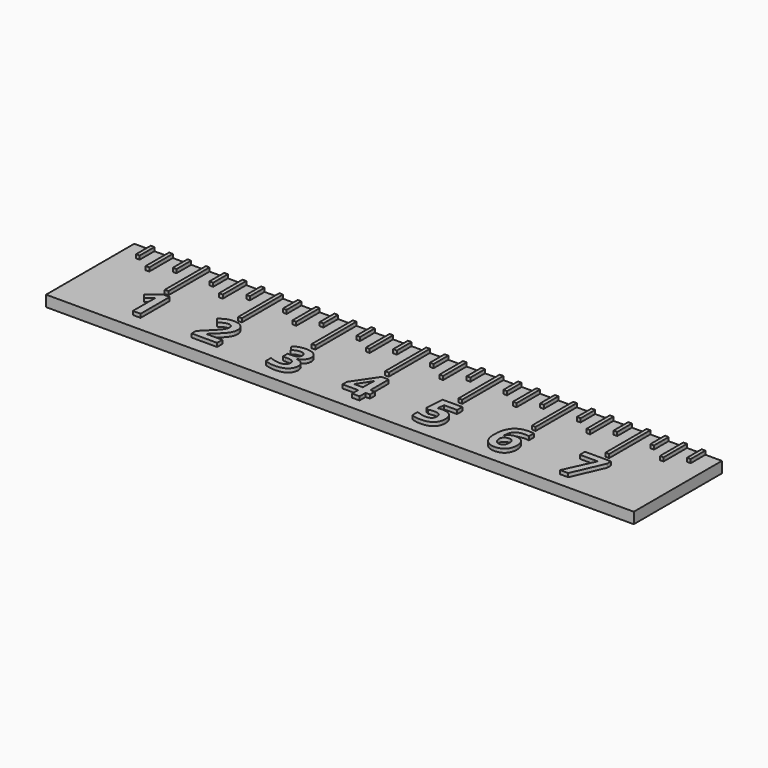
from build123d import *

# Parameters (mm, degrees)
F1_DEPTH     = 3.81
F0_W         = 0.635
F0_H         = 6.35
F0_H_2       = 10.16
F0_H_3       = 17.78
F0_TEXT_SIZE = 17.6388888889
F2_DEPTH     = 5.08


# Not quite as in the source:
# - Text() gives the source's letters only with a copy of the font that has no kerning and outlines rounded to 1/6400 em; it was checked with that copy


with BuildPart() as f1:
    # F0 (on Top) → F1 (new body)
    with BuildSketch(Plane.XY):
        Polygon((-69.85, 29.4929609475), (-75.565, 29.4929609475), (-75.565, -8.6070390525), (127.635, -8.6070390525), (127.635, 29.4929609475), (121.92, 29.4929609475), (121.92, 23.1429609475), (121.285, 23.1429609475), (120.65, 23.1429609475), (120.65, 29.4929609475), (115.57, 29.4929609475), (115.57, 19.3329609475), (114.935, 19.3329609475), (114.3, 19.3329609475), (114.3, 29.4929609475), (109.22, 29.4929609475), (109.22, 23.1429609475), (108.585, 23.1429609475), (107.95, 23.1429609475), (107.95, 29.4929609475), (102.87, 29.4929609475), (102.87, 11.7129609475), (102.235, 11.7129609475), (101.6, 11.7129609475), (101.6, 29.4929609475), (96.52, 29.4929609475), (96.52, 23.1429609475), (95.885, 23.1429609475), (95.25, 23.1429609475), (95.25, 29.4929609475), (90.17, 29.4929609475), (90.17, 19.3329609475), (89.535, 19.3329609475), (88.9, 19.3329609475), (88.9, 29.4929609475), (83.82, 29.4929609475), (83.82, 23.1429609475), (83.185, 23.1429609475), (82.55, 23.1429609475), (82.55, 29.4929609475), (77.47, 29.4929609475), (77.47, 11.7129609475), (76.835, 11.7129609475), (76.2, 11.7129609475), (76.2, 29.4929609475), (71.12, 29.4929609475), (71.12, 23.1429609475), (70.485, 23.1429609475), (69.85, 23.1429609475), (69.85, 29.4929609475), (64.77, 29.4929609475), (64.77, 19.3329609475), (64.135, 19.3329609475), (63.5, 19.3329609475), (63.5, 29.4929609475), (58.42, 29.4929609475), (58.42, 23.1429609475), (57.785, 23.1429609475), (57.15, 23.1429609475), (57.15, 29.4929609475), (52.07, 29.4929609475), (52.07, 11.7129609475), (51.435, 11.7129609475), (50.8, 11.7129609475), (50.8, 29.4929609475), (45.72, 29.4929609475), (45.72, 23.1429609475), (45.085, 23.1429609475), (44.45, 23.1429609475), (44.45, 29.4929609475), (39.37, 29.4929609475), (39.37, 19.3329609475), (38.735, 19.3329609475), (38.1, 19.3329609475), (38.1, 29.4929609475), (33.02, 29.4929609475), (33.02, 23.1429609475), (32.385, 23.1429609475), (31.75, 23.1429609475), (31.75, 29.4929609475), (26.67, 29.4929609475), (26.67, 11.7129609475), (26.035, 11.7129609475), (25.4, 11.7129609475), (25.4, 29.4929609475), (20.32, 29.4929609475), (20.32, 23.1429609475), (19.685, 23.1429609475), (19.05, 23.1429609475), (19.05, 29.4929609475), (13.97, 29.4929609475), (13.97, 19.3329609475), (13.335, 19.3329609475), (12.7, 19.3329609475), (12.7, 29.4929609475), (7.62, 29.4929609475), (7.62, 23.1429609475), (6.985, 23.1429609475), (6.35, 23.1429609475), (6.35, 29.4929609475), (1.27, 29.4929609475), (1.27, 11.7129609475), (0.635, 11.7129609475), (0, 11.7129609475), (0, 29.4929609475), (-5.08, 29.4929609475), (-5.08, 23.1429609475), (-5.715, 23.1429609475), (-6.35, 23.1429609475), (-6.35, 29.4929609475), (-11.43, 29.4929609475), (-11.43, 19.3329609475), (-12.065, 19.3329609475), (-12.7, 19.3329609475), (-12.7, 29.4929609475), (-17.78, 29.4929609475), (-17.78, 23.1429609475), (-18.415, 23.1429609475), (-19.05, 23.1429609475), (-19.05, 29.4929609475), (-24.13, 29.4929609475), (-24.13, 11.7129609475), (-24.765, 11.7129609475), (-25.4, 11.7129609475), (-25.4, 29.4929609475), (-30.48, 29.4929609475), (-30.48, 23.1429609475), (-31.115, 23.1429609475), (-31.75, 23.1429609475), (-31.75, 29.4929609475), (-36.83, 29.4929609475), (-36.83, 19.3329609475), (-37.465, 19.3329609475), (-38.1, 19.3329609475), (-38.1, 29.4929609475), (-43.18, 29.4929609475), (-43.18, 23.1429609475), (-43.815, 23.1429609475), (-44.45, 23.1429609475), (-44.45, 29.4929609475), (-49.53, 29.4929609475), (-49.53, 11.7129609475), (-50.165, 11.7129609475), (-50.8, 11.7129609475), (-50.8, 29.4929609475), (-55.88, 29.4929609475), (-55.88, 23.1429609475), (-56.515, 23.1429609475), (-57.15, 23.1429609475), (-57.15, 29.4929609475), (-62.23, 29.4929609475), (-62.23, 19.3329609475), (-62.865, 19.3329609475), (-63.5, 19.3329609475), (-63.5, 29.4929609475), (-68.58, 29.4929609475), (-68.58, 23.1429609475), (-69.215, 23.1429609475), (-69.85, 23.1429609475), align=None)
        with BuildLine():
            Line((-47.136638159, 9.3029846763), (-47.136638159, -3.2895283446))
            Line((-47.136638159, -3.2895283446), (-49.7990079507, -3.2895283446))
            Line((-49.7990079507, -3.2895283446), (-49.7990079507, 3.9975376277))
            Line((-49.7990079507, 3.9975376277), (-49.7714471868, 5.1936747804))
            Line((-49.7714471868, 5.1936747804), (-49.7301060409, 6.5028110652))
            add(Edge.make_bspline(
                [(-49.7301060409, 6.5028110652), (-50.3915643743, 5.8413527318), (-50.6506355548, 5.6346470027)],
                knots=[0, 0, 0, 1, 1, 1], degree=2))
            Line((-50.6506355548, 5.6346470027), (-52.097575659, 4.4715827665))
            Line((-52.097575659, 4.4715827665), (-53.3819072562, 6.0728631485))
            Line((-53.3819072562, 6.0728631485), (-49.3249628118, 9.3029846763))
            Line((-49.3249628118, 9.3029846763), (-47.136638159, 9.3029846763))
        make_face(mode=Mode.SUBTRACT)
        with BuildLine():
            Line((-20.3797193368, -1.4265028158), (-20.3797193368, -3.6671929199))
            Line((-20.3797193368, -3.6671929199), (-29.1826273229, -3.6671929199))
            Line((-29.1826273229, -3.6671929199), (-29.1826273229, -1.8151095866))
            Line((-29.1826273229, -1.8151095866), (-26.0214077049, 1.3791829481))
            add(Edge.make_bspline(
                [(-26.0214077049, 1.3791829481), (-24.6158087465, 2.8178548231), (-24.1858608299, 3.3732042155)],
                knots=[0, 0, 0, 1, 1, 1], degree=2))
            add(Edge.make_bspline(
                [(-24.1858608299, 3.3732042155), (-23.7559129132, 3.9285536079), (-23.5657436424, 4.4025987467)],
                knots=[0, 0, 0, 1, 1, 1], degree=2))
            add(Edge.make_bspline(
                [(-23.5657436424, 4.4025987467), (-23.3755743715, 4.8766438856), (-23.3755743715, 5.3837619412)],
                knots=[0, 0, 0, 1, 1, 1], degree=2))
            add(Edge.make_bspline(
                [(-23.3755743715, 5.3837619412), (-23.3755743715, 6.1416829481), (-23.7944979827, 6.5123752224)],
                knots=[0, 0, 0, 1, 1, 1], degree=2))
            add(Edge.make_bspline(
                [(-23.7944979827, 6.5123752224), (-24.2134215938, 6.8830674967), (-24.9107089202, 6.8830674967)],
                knots=[0, 0, 0, 1, 1, 1], degree=2))
            add(Edge.make_bspline(
                [(-24.9107089202, 6.8830674967), (-25.6410691632, 6.8830674967), (-26.3300882604, 6.5468261773)],
                knots=[0, 0, 0, 1, 1, 1], degree=2))
            add(Edge.make_bspline(
                [(-26.3300882604, 6.5468261773), (-27.0191073577, 6.2105848579), (-27.7687601354, 5.5904676704)],
                knots=[0, 0, 0, 1, 1, 1], degree=2))
            Line((-27.7687601354, 5.5904676704), (-29.2157002396, 7.3047471842))
            add(Edge.make_bspline(
                [(-29.2157002396, 7.3047471842), (-28.2869024965, 8.0984971842), (-27.6750535382, 8.4250922363)],
                knots=[0, 0, 0, 1, 1, 1], degree=2))
            add(Edge.make_bspline(
                [(-27.6750535382, 8.4250922363), (-27.0632045799, 8.7516872884), (-26.3397345278, 8.9280761773)],
                knots=[0, 0, 0, 1, 1, 1], degree=2))
            add(Edge.make_bspline(
                [(-26.3397345278, 8.9280761773), (-25.6162644757, 9.1044650662), (-24.7205396493, 9.1044650662)],
                knots=[0, 0, 0, 1, 1, 1], degree=2))
            add(Edge.make_bspline(
                [(-24.7205396493, 9.1044650662), (-23.5409389549, 9.1044650662), (-22.6369458993, 8.6745171495)],
                knots=[0, 0, 0, 1, 1, 1], degree=2))
            add(Edge.make_bspline(
                [(-22.6369458993, 8.6745171495), (-21.7329528438, 8.2445692329), (-21.2327249792, 7.4687337294)],
                knots=[0, 0, 0, 1, 1, 1], degree=2))
            add(Edge.make_bspline(
                [(-21.2327249792, 7.4687337294), (-20.7324971146, 6.6928982259), (-20.7324971146, 5.6951985731)],
                knots=[0, 0, 0, 1, 1, 1], degree=2))
            add(Edge.make_bspline(
                [(-20.7324971146, 5.6951985731), (-20.7324971146, 4.8242784342), (-21.0384215938, 4.0622233127)],
                knots=[0, 0, 0, 1, 1, 1], degree=2))
            add(Edge.make_bspline(
                [(-21.0384215938, 4.0622233127), (-21.3443460729, 3.3001681912), (-21.9865118715, 2.4995280002)],
                knots=[0, 0, 0, 1, 1, 1], degree=2))
            add(Edge.make_bspline(
                [(-21.9865118715, 2.4995280002), (-22.6286776702, 1.6988878092), (-24.2464945104, 0.216118712)],
                knots=[0, 0, 0, 1, 1, 1], degree=2))
            Line((-24.2464945104, 0.216118712), (-25.8670674271, -1.307991531))
            Line((-25.8670674271, -1.307991531), (-25.8670674271, -1.4265028158))
            Line((-25.8670674271, -1.4265028158), (-20.3797193368, -1.4265028158))
        make_face(mode=Mode.SUBTRACT)
        with BuildLine():
            add(Edge.make_bspline(
                [(3.7243620052, 7.7445760939), (4.857109401, 6.9522041321), (4.857109401, 5.541093021)],
                knots=[0, 0, 0, 1, 1, 1], degree=2))
            add(Edge.make_bspline(
                [(4.857109401, 5.541093021), (4.857109401, 4.3614923265), (4.1419075781, 3.5346694099)],
                knots=[0, 0, 0, 1, 1, 1], degree=2))
            add(Edge.make_bspline(
                [(4.1419075781, 3.5346694099), (3.4267057552, 2.7078464932), (2.1341059288, 2.3964098612)],
                knots=[0, 0, 0, 1, 1, 1], degree=2))
            Line((2.1341059288, 2.3964098612), (2.1341059288, 2.3468004862))
            add(Edge.make_bspline(
                [(2.1341059288, 2.3468004862), (3.6609722483, 2.1566312154), (4.4436979427, 1.4193807814)],
                knots=[0, 0, 0, 1, 1, 1], degree=2))
            add(Edge.make_bspline(
                [(4.4436979427, 1.4193807814), (5.2264236372, 0.6821303474), (5.2264236372, -0.5663722568)],
                knots=[0, 0, 0, 1, 1, 1], degree=2))
            add(Edge.make_bspline(
                [(5.2264236372, -0.5663722568), (5.2264236372, -2.3826265971), (3.9090191233, -3.39548467)],
                knots=[0, 0, 0, 1, 1, 1], degree=2))
            add(Edge.make_bspline(
                [(3.9090191233, -3.39548467), (2.5916146094, -4.4083427429), (0.1469748524, -4.4083427429)],
                knots=[0, 0, 0, 1, 1, 1], degree=2))
            add(Edge.make_bspline(
                [(0.1469748524, -4.4083427429), (-1.9035459809, -4.4083427429), (-3.4882899045, -3.7275918749)],
                knots=[0, 0, 0, 1, 1, 1], degree=2))
            Line((-3.4882899045, -3.7275918749), (-3.4882899045, -1.4620970832))
            add(Edge.make_bspline(
                [(-3.4882899045, -1.4620970832), (-2.7579296615, -1.8314113193), (-1.8787412934, -2.0642997742)],
                knots=[0, 0, 0, 1, 1, 1], degree=2))
            add(Edge.make_bspline(
                [(-1.8787412934, -2.0642997742), (-0.9995529253, -2.297188229), (-0.139657092, -2.297188229)],
                knots=[0, 0, 0, 1, 1, 1], degree=2))
            add(Edge.make_bspline(
                [(-0.139657092, -2.297188229), (1.1805034983, -2.297188229), (1.8088889149, -1.8493258158)],
                knots=[0, 0, 0, 1, 1, 1], degree=2))
            add(Edge.make_bspline(
                [(1.8088889149, -1.8493258158), (2.4372743316, -1.4014634026), (2.4372743316, -0.4092759026)],
                knots=[0, 0, 0, 1, 1, 1], degree=2))
            add(Edge.make_bspline(
                [(2.4372743316, -0.4092759026), (2.4372743316, 0.4754246182), (1.7138042795, 0.8461168925)],
                knots=[0, 0, 0, 1, 1, 1], degree=2))
            add(Edge.make_bspline(
                [(1.7138042795, 0.8461168925), (0.9903342274, 1.2168091668), (-0.5944096962, 1.2168091668)],
                knots=[0, 0, 0, 1, 1, 1], degree=2))
            Line((-0.5944096962, 1.2168091668), (-1.5507682031, 1.2168091668))
            Line((-1.5507682031, 1.2168091668), (-1.5507682031, 3.259061771))
            Line((-1.5507682031, 3.259061771), (-0.5778732378, 3.259061771))
            add(Edge.make_bspline(
                [(-0.5778732378, 3.259061771), (0.8856033247, 3.259061771), (1.5622200781, 3.642156389)],
                knots=[0, 0, 0, 1, 1, 1], degree=2))
            add(Edge.make_bspline(
                [(1.5622200781, 3.642156389), (2.2388368316, 4.0252510071), (2.2388368316, 4.9540487501)],
                knots=[0, 0, 0, 1, 1, 1], degree=2))
            add(Edge.make_bspline(
                [(2.2388368316, 4.9540487501), (2.2388368316, 6.384452396), (0.4473871788, 6.384452396)],
                knots=[0, 0, 0, 1, 1, 1], degree=2))
            add(Edge.make_bspline(
                [(0.4473871788, 6.384452396), (-0.1727300087, 6.384452396), (-0.8148958073, 6.1777466668)],
                knots=[0, 0, 0, 1, 1, 1], degree=2))
            add(Edge.make_bspline(
                [(-0.8148958073, 6.1777466668), (-1.4570616059, 5.9710409376), (-2.2397873003, 5.4639228821)],
                knots=[0, 0, 0, 1, 1, 1], degree=2))
            Line((-2.2397873003, 5.4639228821), (-3.4717534462, 7.2967136807))
            add(Edge.make_bspline(
                [(-3.4717534462, 7.2967136807), (-1.7492057031, 8.5369480557), (0.6375564497, 8.5369480557)],
                knots=[0, 0, 0, 1, 1, 1], degree=2))
            add(Edge.make_bspline(
                [(0.6375564497, 8.5369480557), (2.5916146094, 8.5369480557), (3.7243620052, 7.7445760939)],
                knots=[0, 0, 0, 1, 1, 1], degree=2))
        make_face(mode=Mode.SUBTRACT)
        Polygon((30.7129252507, 0.6035627079), (30.7129252507, -1.4634945838), (29.1970832368, -1.4634945838), (29.1970832368, -4.0734989241), (26.5953471257, -4.0734989241), (26.5953471257, -1.4634945838), (21.2209981673, -1.4634945838), (21.2209981673, 0.3885887495), (26.7441752507, 8.5190140968), (29.1970832368, 8.5190140968), (29.1970832368, 0.6035627079), align=None, mode=Mode.SUBTRACT)
        with BuildLine():
            add(Edge.make_bspline(
                [(50.3075025767, 3.7392927248), (50.8339131669, 3.8605600859), (51.6083706322, 3.8605600859)],
                knots=[0, 0, 0, 1, 1, 1], degree=2))
            add(Edge.make_bspline(
                [(51.6083706322, 3.8605600859), (53.4328932017, 3.8605600859), (54.5146531843, 2.8352996692)],
                knots=[0, 0, 0, 1, 1, 1], degree=2))
            add(Edge.make_bspline(
                [(54.5146531843, 2.8352996692), (55.5964131669, 1.8100392525), (55.5964131669, 0.0268578289)],
                knots=[0, 0, 0, 1, 1, 1], degree=2))
            add(Edge.make_bspline(
                [(55.5964131669, 0.0268578289), (55.5964131669, -2.0815406086), (54.2955451114, -3.2198001572)],
                knots=[0, 0, 0, 1, 1, 1], degree=2))
            add(Edge.make_bspline(
                [(54.2955451114, -3.2198001572), (52.9946770558, -4.3580597058), (50.5748419864, -4.3580597058)],
                knots=[0, 0, 0, 1, 1, 1], degree=2))
            add(Edge.make_bspline(
                [(50.5748419864, -4.3580597058), (48.4719557017, -4.3580597058), (47.1821119517, -3.6773088377)],
                knots=[0, 0, 0, 1, 1, 1], degree=2))
            Line((47.1821119517, -3.6773088377), (47.1821119517, -1.375985053))
            add(Edge.make_bspline(
                [(47.1821119517, -1.375985053), (47.8601067433, -1.73703106), (48.7654778371, -1.9657854002)],
                knots=[0, 0, 0, 1, 1, 1], degree=2))
            add(Edge.make_bspline(
                [(48.7654778371, -1.9657854002), (49.6708489308, -2.1945397405), (50.4783793128, -2.1945397405)],
                knots=[0, 0, 0, 1, 1, 1], degree=2))
            add(Edge.make_bspline(
                [(50.4783793128, -2.1945397405), (52.9175069169, -2.1945397405), (52.9175069169, -0.1963843586)],
                knots=[0, 0, 0, 1, 1, 1], degree=2))
            add(Edge.make_bspline(
                [(52.9175069169, -0.1963843586), (52.9175069169, 1.7080644262), (50.3929409447, 1.7080644262)],
                knots=[0, 0, 0, 1, 1, 1], degree=2))
            add(Edge.make_bspline(
                [(50.3929409447, 1.7080644262), (49.9381883406, 1.7080644262), (49.3869730628, 1.6171139053)],
                knots=[0, 0, 0, 1, 1, 1], degree=2))
            add(Edge.make_bspline(
                [(49.3869730628, 1.6171139053), (48.835757785, 1.5261633845), (48.4912482364, 1.4214324817)],
                knots=[0, 0, 0, 1, 1, 1], degree=2))
            Line((48.4912482364, 1.4214324817), (47.4301588267, 1.9919402942))
            Line((47.4301588267, 1.9919402942), (47.9042039656, 8.4080861275))
            Line((47.9042039656, 8.4080861275), (54.7337612572, 8.4080861275))
            Line((54.7337612572, 8.4080861275), (54.7337612572, 6.150859565))
            Line((54.7337612572, 6.150859565), (50.2386006669, 6.150859565))
            Line((50.2386006669, 6.150859565), (50.0070902503, 3.6786590442))
            Line((50.0070902503, 3.6786590442), (50.3075025767, 3.7392927248))
        make_face(mode=Mode.SUBTRACT)
        with BuildLine():
            add(Edge.make_bspline(
                [(72.0270052565, -1.835879369), (71.463387635, -0.595644994), (71.463387635, 1.1544635129)],
                knots=[0, 0, 0, 1, 1, 1], degree=2))
            add(Edge.make_bspline(
                [(71.463387635, 1.1544635129), (71.463387635, 4.8917030963), (73.043997444, 6.7176037039)],
                knots=[0, 0, 0, 1, 1, 1], degree=2))
            add(Edge.make_bspline(
                [(73.043997444, 6.7176037039), (74.624607253, 8.5435043116), (77.7775586419, 8.5435043116)],
                knots=[0, 0, 0, 1, 1, 1], degree=2))
            add(Edge.make_bspline(
                [(77.7775586419, 8.5435043116), (78.8524284336, 8.5435043116), (79.4642773919, 8.4139687213)],
                knots=[0, 0, 0, 1, 1, 1], degree=2))
            Line((79.4642773919, 8.4139687213), (79.4642773919, 6.2862777491))
            add(Edge.make_bspline(
                [(79.4642773919, 6.2862777491), (78.6980881558, 6.4599105616), (77.948435378, 6.4599105616)],
                knots=[0, 0, 0, 1, 1, 1], degree=2))
            add(Edge.make_bspline(
                [(77.948435378, 6.4599105616), (76.5786654128, 6.4599105616), (75.7132574266, 6.0464991032)],
                knots=[0, 0, 0, 1, 1, 1], degree=2))
            add(Edge.make_bspline(
                [(75.7132574266, 6.0464991032), (74.8478494405, 5.6330876449), (74.4179015239, 4.8228011866)],
                knots=[0, 0, 0, 1, 1, 1], degree=2))
            add(Edge.make_bspline(
                [(74.4179015239, 4.8228011866), (73.9879536072, 4.0125147282), (73.9107834683, 2.5242334782)],
                knots=[0, 0, 0, 1, 1, 1], degree=2))
            Line((73.9107834683, 2.5242334782), (74.0210265239, 2.5242334782))
            add(Edge.make_bspline(
                [(74.0210265239, 2.5242334782), (74.8754102044, 3.9877100407), (76.7522982253, 3.9877100407)],
                knots=[0, 0, 0, 1, 1, 1], degree=2))
            add(Edge.make_bspline(
                [(76.7522982253, 3.9877100407), (78.4390169753, 3.9877100407), (79.3953754822, 2.9279986692)],
                knots=[0, 0, 0, 1, 1, 1], degree=2))
            add(Edge.make_bspline(
                [(79.3953754822, 2.9279986692), (80.3517339891, 1.8682872977), (80.3517339891, -0.000332494)],
                knots=[0, 0, 0, 1, 1, 1], degree=2))
            add(Edge.make_bspline(
                [(80.3517339891, -0.000332494), (80.3517339891, -2.0150243343), (79.2148524787, -3.1918689523)],
                knots=[0, 0, 0, 1, 1, 1], degree=2))
            add(Edge.make_bspline(
                [(79.2148524787, -3.1918689523), (78.0779709683, -4.3687135704), (76.063279128, -4.3687135704)],
                knots=[0, 0, 0, 1, 1, 1], degree=2))
            add(Edge.make_bspline(
                [(76.063279128, -4.3687135704), (74.6687044753, -4.3687135704), (73.6296636766, -3.7224136572)],
                knots=[0, 0, 0, 1, 1, 1], degree=2))
            add(Edge.make_bspline(
                [(73.6296636766, -3.7224136572), (72.590622878, -3.076113744), (72.0270052565, -1.835879369)],
                knots=[0, 0, 0, 1, 1, 1], degree=2))
        make_face(mode=Mode.SUBTRACT)
        Polygon((101.217452068, -3.9223459687), (98.4255466861, -3.9223459687), (103.1549737694, 6.4129404896), (96.9455336652, 6.4129404896), (96.9455336652, 8.6536305938), (105.979952068, 8.6536305938), (105.979952068, 6.9806922257), align=None, mode=Mode.SUBTRACT)
    extrude(amount=F1_DEPTH)


with BuildPart() as f1b:
    # F0 (on Top) → F1, piece 2 (new body)
    with BuildSketch(Plane.XY):
        with BuildLine():
            Line((23.5636630979, 0.6035627079), (26.5953471257, 0.6035627079))
            Line((26.5953471257, 0.6035627079), (26.5953471257, 2.7395219093))
            add(Edge.make_bspline(
                [(26.5953471257, 2.7395219093), (26.5953471257, 3.2742007287), (26.6394443479, 4.289814878)],
                knots=[0, 0, 0, 1, 1, 1], degree=2))
            add(Edge.make_bspline(
                [(26.6394443479, 4.289814878), (26.6835415701, 5.3054290273), (26.7083462576, 5.4707936106)],
                knots=[0, 0, 0, 1, 1, 1], degree=2))
            Line((26.7083462576, 5.4707936106), (26.6394443479, 5.4707936106))
            add(Edge.make_bspline(
                [(26.6394443479, 5.4707936106), (26.3197394868, 4.7624819787), (25.8732551118, 4.0927554162)],
                knots=[0, 0, 0, 1, 1, 1], degree=2))
            Line((25.8732551118, 4.0927554162), (23.5636630979, 0.6035627079))
        make_face()
    extrude(amount=F1_DEPTH)


with BuildPart() as f1c:
    # F0 (on Top) → F1, piece 3 (new body)
    with BuildSketch(Plane.XY):
        with BuildLine():
            add(Edge.make_bspline(
                [(74.6452778259, -1.5340890044), (75.18409076, -2.2410225982), (76.0109136766, -2.2410225982)],
                knots=[0, 0, 0, 1, 1, 1], degree=2))
            add(Edge.make_bspline(
                [(76.0109136766, -2.2410225982), (76.8625412808, -2.2410225982), (77.3200499614, -1.6677587093)],
                knots=[0, 0, 0, 1, 1, 1], degree=2))
            add(Edge.make_bspline(
                [(77.3200499614, -1.6677587093), (77.7775586419, -1.0944948204), (77.7775586419, -0.0361614871)],
                knots=[0, 0, 0, 1, 1, 1], degree=2))
            add(Edge.make_bspline(
                [(77.7775586419, -0.0361614871), (77.7775586419, 0.8871241032), (77.3503668016, 1.4162907699)],
                knots=[0, 0, 0, 1, 1, 1], degree=2))
            add(Edge.make_bspline(
                [(77.3503668016, 1.4162907699), (76.9231749614, 1.9454574366), (76.063279128, 1.9454574366)],
                knots=[0, 0, 0, 1, 1, 1], degree=2))
            add(Edge.make_bspline(
                [(76.063279128, 1.9454574366), (75.2529926697, 1.9454574366), (74.6797287808, 1.4204248845)],
                knots=[0, 0, 0, 1, 1, 1], degree=2))
            add(Edge.make_bspline(
                [(74.6797287808, 1.4204248845), (74.1064648919, 0.8953923324), (74.1064648919, 0.198105006)],
                knots=[0, 0, 0, 1, 1, 1], degree=2))
            add(Edge.make_bspline(
                [(74.1064648919, 0.198105006), (74.1064648919, -0.8271554107), (74.6452778259, -1.5340890044)],
                knots=[0, 0, 0, 1, 1, 1], degree=2))
        make_face()
    extrude(amount=F1_DEPTH)


with BuildPart() as f2:
    # F0 (on Top) → F2 (new body)
    with BuildSketch(Plane.XY):
        with Locations((-68.8975, 26.3179609475)):
            Rectangle(F0_W, F0_H)
        with Locations((-69.5325, 26.3179609475)):
            Rectangle(F0_W, F0_H)
        with Locations((-63.1825, 24.4129609475)):
            Rectangle(F0_W, F0_H_2)
        with Locations((-62.5475, 24.4129609475)):
            Rectangle(F0_W, F0_H_2)
        with Locations((-56.8325, 26.3179609475)):
            Rectangle(F0_W, F0_H)
        with Locations((-56.1975, 26.3179609475)):
            Rectangle(F0_W, F0_H)
        with Locations((-50.4825, 20.6029609475)):
            Rectangle(F0_W, F0_H_3)
        with Locations((-49.8475, 20.6029609475)):
            Rectangle(F0_W, F0_H_3)
        with Locations((-44.1325, 26.3179609475)):
            Rectangle(F0_W, F0_H)
        with Locations((-37.1475, 24.4129609475)):
            Rectangle(F0_W, F0_H_2)
        with Locations((-31.4325, 26.3179609475)):
            Rectangle(F0_W, F0_H)
        with Locations((-30.7975, 26.3179609475)):
            Rectangle(F0_W, F0_H)
        with Locations((-43.4975, 26.3179609475)):
            Rectangle(F0_W, F0_H)
        with Locations((-37.7825, 24.4129609475)):
            Rectangle(F0_W, F0_H_2)
        with Locations((-25.0825, 20.6029609475)):
            Rectangle(F0_W, F0_H_3)
        with Locations((-24.4475, 20.6029609475)):
            Rectangle(F0_W, F0_H_3)
        with Locations((-18.7325, 26.3179609475)):
            Rectangle(F0_W, F0_H)
        with Locations((-18.0975, 26.3179609475)):
            Rectangle(F0_W, F0_H)
        with Locations((-11.7475, 24.4129609475)):
            Rectangle(F0_W, F0_H_2)
        with Locations((-6.0325, 26.3179609475)):
            Rectangle(F0_W, F0_H)
        with Locations((-12.3825, 24.4129609475)):
            Rectangle(F0_W, F0_H_2)
        with Locations((-5.3975, 26.3179609475)):
            Rectangle(F0_W, F0_H)
        with Locations((0.3175, 20.6029609475)):
            Rectangle(F0_W, F0_H_3)
        with Locations((0.9525, 20.6029609475)):
            Rectangle(F0_W, F0_H_3)
        with Locations((6.6675, 26.3179609475)):
            Rectangle(F0_W, F0_H)
        with Locations((7.3025, 26.3179609475)):
            Rectangle(F0_W, F0_H)
        with Locations((13.0175, 24.4129609475)):
            Rectangle(F0_W, F0_H_2)
        with Locations((13.6525, 24.4129609475)):
            Rectangle(F0_W, F0_H_2)
        with Locations((20.0025, 26.3179609475)):
            Rectangle(F0_W, F0_H)
        with Locations((19.3675, 26.3179609475)):
            Rectangle(F0_W, F0_H)
        with Locations((26.3525, 20.6029609475)):
            Rectangle(F0_W, F0_H_3)
        with Locations((25.7175, 20.6029609475)):
            Rectangle(F0_W, F0_H_3)
        with Locations((32.0675, 26.3179609475)):
            Rectangle(F0_W, F0_H)
        with Locations((32.7025, 26.3179609475)):
            Rectangle(F0_W, F0_H)
        with Locations((38.4175, 24.4129609475)):
            Rectangle(F0_W, F0_H_2)
        with Locations((39.0525, 24.4129609475)):
            Rectangle(F0_W, F0_H_2)
        with Locations((44.7675, 26.3179609475)):
            Rectangle(F0_W, F0_H)
        with Locations((45.4025, 26.3179609475)):
            Rectangle(F0_W, F0_H)
        with Locations((51.1175, 20.6029609475)):
            Rectangle(F0_W, F0_H_3)
        with Locations((51.7525, 20.6029609475)):
            Rectangle(F0_W, F0_H_3)
        with Locations((57.4675, 26.3179609475)):
            Rectangle(F0_W, F0_H)
        with Locations((63.8175, 24.4129609475)):
            Rectangle(F0_W, F0_H_2)
        with Locations((58.1025, 26.3179609475)):
            Rectangle(F0_W, F0_H)
        with Locations((64.4525, 24.4129609475)):
            Rectangle(F0_W, F0_H_2)
        with Locations((70.1675, 26.3179609475)):
            Rectangle(F0_W, F0_H)
        with Locations((70.8025, 26.3179609475)):
            Rectangle(F0_W, F0_H)
        with Locations((76.5175, 20.6029609475)):
            Rectangle(F0_W, F0_H_3)
        with Locations((77.1525, 20.6029609475)):
            Rectangle(F0_W, F0_H_3)
        with Locations((82.8675, 26.3179609475)):
            Rectangle(F0_W, F0_H)
        with Locations((83.5025, 26.3179609475)):
            Rectangle(F0_W, F0_H)
        with Locations((89.2175, 24.4129609475)):
            Rectangle(F0_W, F0_H_2)
        with Locations((89.8525, 24.4129609475)):
            Rectangle(F0_W, F0_H_2)
        with Locations((95.5675, 26.3179609475)):
            Rectangle(F0_W, F0_H)
        with Locations((96.2025, 26.3179609475)):
            Rectangle(F0_W, F0_H)
        with Locations((101.9175, 20.6029609475)):
            Rectangle(F0_W, F0_H_3)
        with Locations((102.5525, 20.6029609475)):
            Rectangle(F0_W, F0_H_3)
        with Locations((108.2675, 26.3179609475)):
            Rectangle(F0_W, F0_H)
        with Locations((108.9025, 26.3179609475)):
            Rectangle(F0_W, F0_H)
        with Locations((114.6175, 24.4129609475)):
            Rectangle(F0_W, F0_H_2)
        with Locations((115.2525, 24.4129609475)):
            Rectangle(F0_W, F0_H_2)
        with Locations((120.9675, 26.3179609475)):
            Rectangle(F0_W, F0_H)
        with Locations((121.6025, 26.3179609475)):
            Rectangle(F0_W, F0_H)
        with Locations((-29.8881828785, -3.6671929199)):
            Text('2', F0_TEXT_SIZE, font='Open Sans', font_style=FontStyle.BOLD, text_align=(TextAlign.LEFT, TextAlign.BOTTOM))
        with Locations((-54.4237041312, -3.2895283446)):
            Text('1', F0_TEXT_SIZE, font='Open Sans', font_style=FontStyle.BOLD, text_align=(TextAlign.LEFT, TextAlign.BOTTOM))
        with Locations((-4.1607725434, -4.2347099304)):
            Text('3', F0_TEXT_SIZE, font='Open Sans', font_style=FontStyle.BOLD, text_align=(TextAlign.LEFT, TextAlign.BOTTOM))
        with Locations((20.9205858409, -4.0734989241)):
            Text('4', F0_TEXT_SIZE, font='Open Sans', font_style=FontStyle.BOLD, text_align=(TextAlign.LEFT, TextAlign.BOTTOM))
        with Locations((46.3194600419, -4.1844268933)):
            Text('5', F0_TEXT_SIZE, font='Open Sans', font_style=FontStyle.BOLD, text_align=(TextAlign.LEFT, TextAlign.BOTTOM))
        with Locations((70.8432704475, -4.1950807579)):
            Text('6', F0_TEXT_SIZE, font='Open Sans', font_style=FontStyle.BOLD, text_align=(TextAlign.LEFT, TextAlign.BOTTOM))
        with Locations((96.4714885263, -3.9223459687)):
            Text('7', F0_TEXT_SIZE, font='Open Sans', font_style=FontStyle.BOLD, text_align=(TextAlign.LEFT, TextAlign.BOTTOM))
    extrude(amount=F2_DEPTH)


solid = Compound([f1.part, f1b.part, f1c.part, f2.part])
